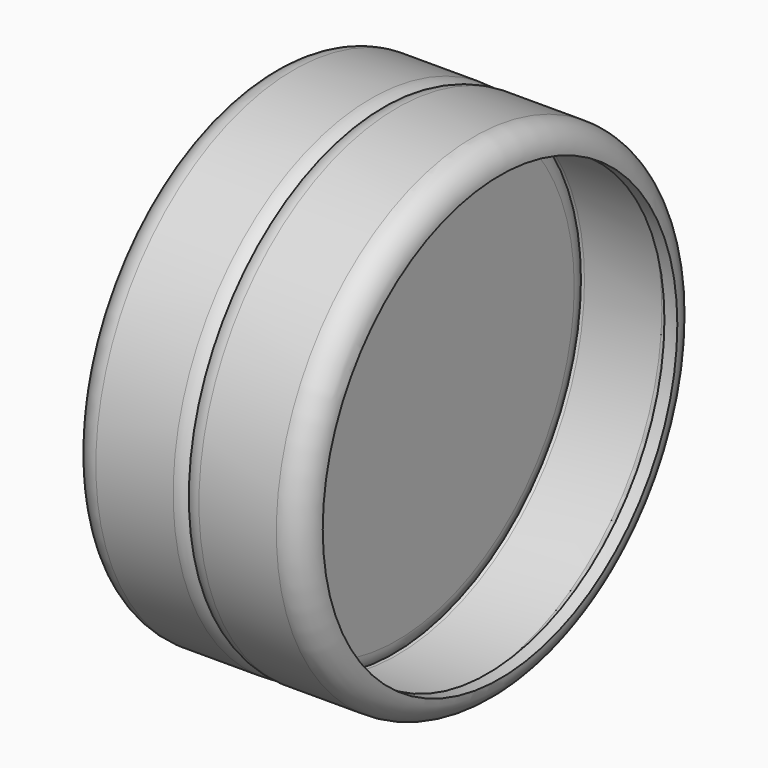
from build123d import *

# Parameters (mm, degrees)
F0_R     = 48.7426
F1_DEPTH = 25.4
F2_R     = 5.08
F3_T     = -2.54


# Not quite as in the source:
# - a shell that OpenCascade refuses in one call is made with other operations: the cavity is built on its own and cut out


with BuildPart() as f1:
    # F0 (on Right) → F1 (new body)
    with BuildSketch(Plane.YZ):
        Circle(F0_R)
    extrude(amount=F1_DEPTH)

    # F2
    f2_edges = [f1.edges().sort_by_distance(p)[0] for p in [
        (12.7, 48.7426, 0),
        (0, -48.7426, 0),
        (25.4, -48.7426, 0),
    ]]
    fillet(f2_edges, radius=F2_R)

    # F3: a shell. OpenCascade refuses it in one call, so the cavity is built on its own and cut out:
    # the body offset inwards by the wall thickness, plus a prism from it out through each open face.
    f3_core = offset(f1.part, amount=F3_T, mode=Mode.PRIVATE)
    f3_exits = [f3_core.faces().sort_by_distance(p)[0] for p in [
        (2.54, 0, 0),
    ]]
    add(f3_core, mode=Mode.SUBTRACT)
    extrude(f3_exits, amount=-F3_T, mode=Mode.SUBTRACT)

    # F4: F1 across face


with BuildPart() as f1_1:
    add(f1.part)
    add(f1.part.mirror(Plane(origin=(22.86, 0, 0), x_dir=(0, -1, 0), z_dir=(-1, 0, 0))))


solid = f1_1.part
